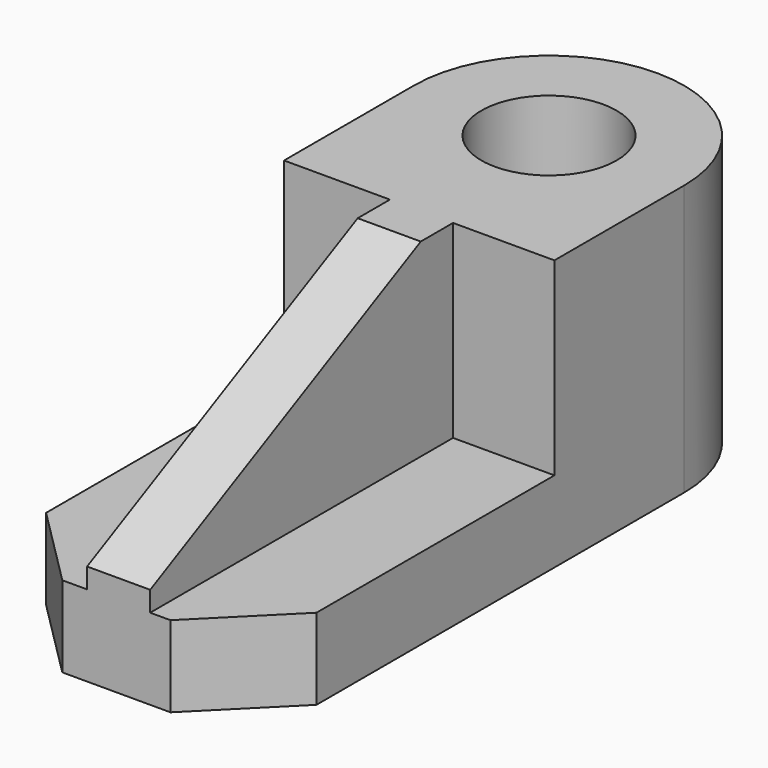
from build123d import *

# Parameters (mm, degrees)
F1_DEPTH  = 9
F2_W      = 7
F2_H      = 42
F3_DEPTH  = 21
F5_DEPTH  = 25
F7_DEPTH  = 30
F8_DEPTH  = 21
F9_R      = 7.5
F10_DEPTH = 30


with BuildPart() as f1:
    # F0 (on Top) → F1 (new body)
    with BuildSketch(Plane.XY):
        Polygon((15, 30), (-15, 30), (-15, -21), (-6, -30), (6, -30), (15, -21), align=None)
    extrude(amount=F1_DEPTH)

    # F2 (on face) → F3 (join)
    with BuildSketch(Plane.XY.offset(9)):
        with Locations((0.25, -9)):
            Rectangle(F2_W, F2_H)
    extrude(amount=F3_DEPTH)

    # F4 (on face) → F5 (cut)
    with BuildSketch(Plane(origin=(-3.25, 0, 0), x_dir=(0, -1, 0), z_dir=(-1, 0, 0))):
        Polygon((30, 30), (-7.5259371102, 30), (30, 11.2370314449), align=None)
    extrude(amount=-F5_DEPTH, mode=Mode.SUBTRACT)

    # F0 (on Top) → F7 (join)
    with BuildSketch(Plane.XY):
        with BuildLine():
            ThreePointArc((15, 30), (0, 45), (-15, 30))
            Line((-15, 30), (15, 30))
        make_face()
    extrude(amount=F7_DEPTH)

    # F6 (on face) → F8 (join)
    with BuildSketch(Plane.XY.offset(9)):
        Polygon((3.75, 12), (15, 12), (15, 30), (-15, 30), (-15, 12), (-3.25, 12), align=None)
    extrude(amount=F8_DEPTH)

    # F9 (on face) → F10 (cut)
    with BuildSketch(Plane.XY.offset(30)):
        with Locations((0, 30)):
            Circle(F9_R)
    extrude(amount=-F10_DEPTH, mode=Mode.SUBTRACT)


solid = f1.part
